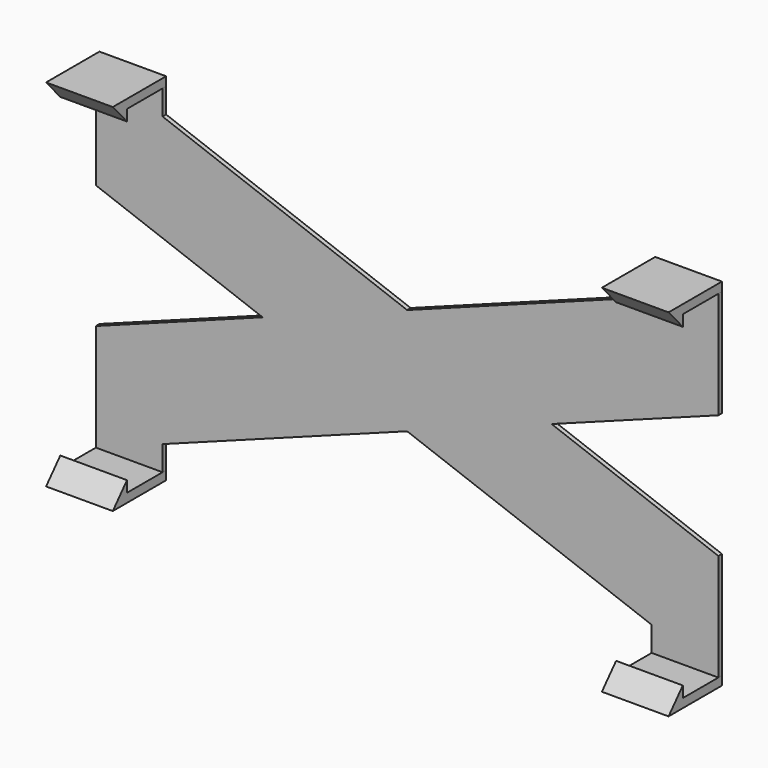
from build123d import *

# Parameters (mm, degrees)
F1_DEPTH  = 1
F0_W      = 15
F0_H      = 2
F2_DEPTH  = 11
F5_DEPTH  = 15
F7_DEPTH  = 15
F9_DEPTH  = 15
F11_DEPTH = 15


# Not quite as in the source:
# - a feature of the source that left no trace in its solid (it failed there, or was rolled back) is left out


with BuildPart() as f1:
    # F0 (on Front) → F1 (new body)
    with BuildSketch(Plane.XZ):
        Polygon((-55, 38), (-70, 38), (-70, 13.9285714286), (-32.5, 0), (-70, -13.9285714286), (-70, -38), (-55, -38), (-55, -32.4285714286), (0, -12), (55, -32.4285714286), (55, -38), (70, -38), (70, -13.9285714286), (32.5, 0), (70, 13.9285714286), (70, 38), (55, 38), (55, 32.4285714286), (0, 12), (-55, 32.4285714286), align=None)
    extrude(amount=F1_DEPTH)


with BuildPart() as f2:
    # F0 (on Front) → F2 (new body)
    with BuildSketch(Plane.XZ):
        with Locations((62.5, 39)):
            Rectangle(F0_W, F0_H)
    extrude(amount=F2_DEPTH)

    # F4 (on face) → F5 (join)
    with BuildSketch(Plane.YZ.offset(70)):
        Polygon((-11, 35.5), (-11, 38), (-11, 40), (-15, 40), align=None)
    extrude(amount=-F5_DEPTH)


with BuildPart() as f2b:
    # F0 (on Front) → F2, piece 2 (new body)
    with BuildSketch(Plane.XZ):
        with Locations((-62.5, 39)):
            Rectangle(F0_W, F0_H)
    extrude(amount=F2_DEPTH)

    # F6 (on face) → F7 (join)
    with BuildSketch(Plane(origin=(-70, 0, 0), x_dir=(0, -1, 0), z_dir=(-1, 0, 0))):
        Polygon((15, 40), (11, 40), (11, 38), (11, 35.5), align=None)
    extrude(amount=-F7_DEPTH)


with BuildPart() as f2c:
    # F0 (on Front) → F2, piece 3 (new body)
    with BuildSketch(Plane.XZ):
        with Locations((-62.5, -39)):
            Rectangle(F0_W, F0_H)
    extrude(amount=F2_DEPTH)

    # F10 (on face) → F11 (join)
    with BuildSketch(Plane(origin=(-70, 0, 0), x_dir=(0, -1, 0), z_dir=(-1, 0, 0))):
        Polygon((11, -35.5), (11, -40), (15, -40), align=None)
    extrude(amount=-F11_DEPTH)


with BuildPart() as f2d:
    # F0 (on Front) → F2, piece 4 (new body)
    with BuildSketch(Plane.XZ):
        with Locations((62.5, -39)):
            Rectangle(F0_W, F0_H)
    extrude(amount=F2_DEPTH)

    # F8 (on face) → F9 (join)
    with BuildSketch(Plane.YZ.offset(70)):
        Polygon((-15, -40), (-11, -40), (-11, -35.5), align=None)
    extrude(amount=-F9_DEPTH)


solid = Compound([f1.part, f2.part, f2b.part, f2c.part, f2d.part])
